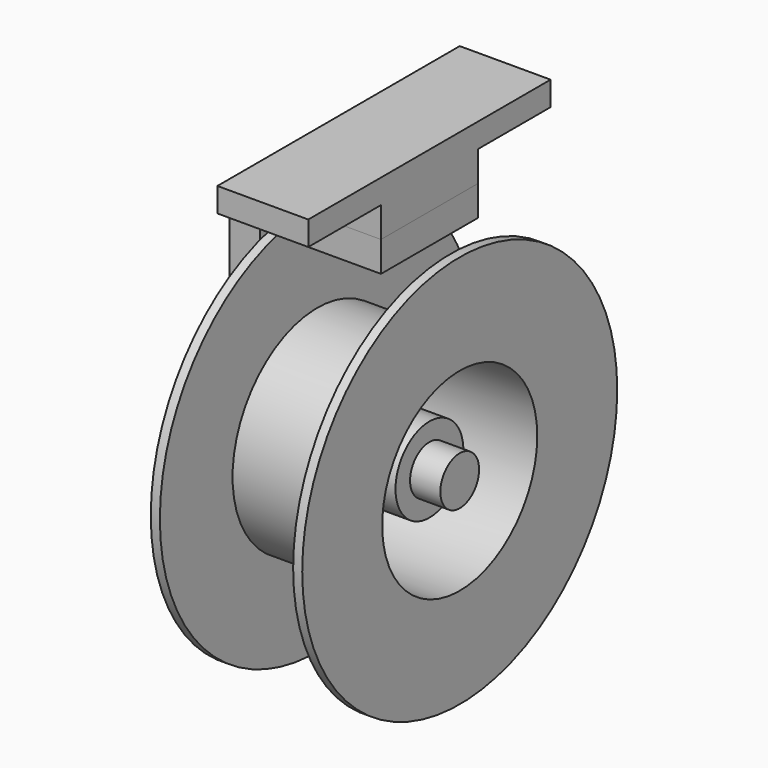
from build123d import *

# Parameters (mm, degrees)
F0_R      = 32.5
F1_DEPTH  = 12.5
F3_DEPTH  = 10
F2_W      = 7.5
F2_H      = 4
F4_DEPTH  = 25
F5_W      = 15
F5_H      = 20
F6_DEPTH  = 9
F7_R      = 4
F8_DEPTH  = 25
F9_START  = -1.5
F7_R_2    = 32.5
F7_R_3    = 17.5
F9_DEPTH  = 22
F7_R_4    = 16
F10_DEPTH = 25
F11_SIZE  = 5
F13_START = -0.5
F12_R     = 16
F12_R_2   = 14
F13_DEPTH = 2
F14_START = -2.5
F12_R_3   = 7
F14_DEPTH = 2.5
F15_DEPTH = 20
F16_DEPTH = 25


with BuildPart() as f1:
    # F0 (on Right) → F1 (new body, symmetric)
    with BuildSketch(Plane.YZ):
        Circle(F0_R)
    extrude(amount=F1_DEPTH, both=True)

    # F7 (on face) → F9 (cut)
    with BuildSketch(Plane.YZ.offset(12.5).offset(F9_START)):
        Circle(F7_R_2)
        Circle(F7_R_3, mode=Mode.SUBTRACT)
    extrude(amount=-F9_DEPTH, mode=Mode.SUBTRACT)

    # F7 (on face) → F10 (cut)
    with BuildSketch(Plane.YZ.offset(12.5)):
        Circle(F7_R_4)
        Circle(F7_R, mode=Mode.SUBTRACT)
        Circle(F7_R)
    extrude(amount=-F10_DEPTH, mode=Mode.SUBTRACT)

    # F12 (on face) → F13 (join)
    with BuildSketch(Plane(origin=(-12.5, 0, 0), x_dir=(0, -1, 0), z_dir=(-1, 0, 0)).offset(F13_START)):
        Circle(F12_R)
        Circle(F12_R_2, mode=Mode.SUBTRACT)
    extrude(amount=-F13_DEPTH)

    # F12 (on face) → F14 (join)
    with BuildSketch(Plane(origin=(-12.5, 0, 0), x_dir=(0, -1, 0), z_dir=(-1, 0, 0)).offset(F14_START)):
        Circle(F12_R)
        Circle(F12_R_2, mode=Mode.SUBTRACT)
        Circle(F12_R_2)
        Circle(F12_R_3, mode=Mode.SUBTRACT)
        Circle(F12_R_3)
    extrude(amount=-F14_DEPTH)

    # F12 (on face) → F15 (join)
    with BuildSketch(Plane(origin=(-12.5, 0, 0), x_dir=(0, -1, 0), z_dir=(-1, 0, 0))):
        Circle(F12_R_3)
    extrude(amount=-F15_DEPTH)

    # F7 (on face) → F16 (cut)
    with BuildSketch(Plane.YZ.offset(12.5)):
        Circle(F7_R)
    extrude(amount=-F16_DEPTH, mode=Mode.SUBTRACT)


with BuildPart() as f3:
    # F2 (on Front) → F3 (new body, symmetric)
    with BuildSketch(Plane.XZ):
        Polygon((-12.5, -12.5), (-12.5, 32.5), (7.5, 32.5), (7.5, 37.5000014901), (-17.5, 37.5000014901), (-17.5, -12.5), align=None)
    extrude(amount=F3_DEPTH, both=True)

    # F11
    f11_edges = [f3.edges().sort_by_distance(p)[0] for p in [
        (-15, 10, -12.5),
        (-15, -10, -12.5),
    ]]
    chamfer(f11_edges, length=F11_SIZE)


with BuildPart() as f4:
    # F2 (on Front) → F4 (new body, symmetric)
    with BuildSketch(Plane.XZ):
        with Locations((-3.75, 44.5000014901)):
            Rectangle(F2_W, F2_H)
        with Locations((3.75, 44.5000014901)):
            Rectangle(F2_W, F2_H)
    extrude(amount=F4_DEPTH, both=True)

    # F5 (on face) → F6 (join, through all)
    with BuildSketch(Plane.XY.offset(46.5000014901)):
        Rectangle(F5_W, F5_H)
    extrude(amount=-F6_DEPTH)


with BuildPart() as f8:
    # F7 (on face) → F8 (new body, through all)
    with BuildSketch(Plane.YZ.offset(12.5)):
        Circle(F7_R)
    extrude(amount=-F8_DEPTH)


solid = Compound([f1.part, f3.part, f4.part, f8.part])
